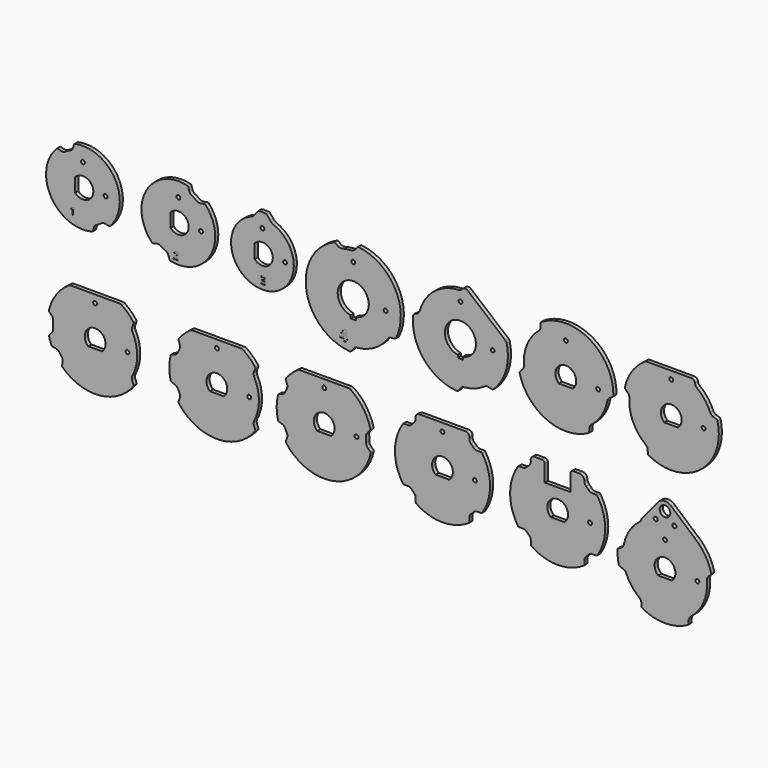
from build123d import *

# Parameters (mm, degrees)
F0_R           = 1.5
F1_DEPTH       = 1.5
F0_R_2         = 1.525
F0_R_3         = 4.1
F2_TEXT_SIZE   = 7.3750813802
F2_TEXT_SIZE_2 = 7.6333681742
F2_TEXT_SIZE_3 = 7.6956219143
F2_TEXT_SIZE_4 = 11.4732318454
F3_DEPTH       = 0.2


# Not quite as in the source:
# - ends of sketch curves that miss each other by under 0.0002 mm in the source are joined
# - Text() gives the source's letters only with a copy of the font that has no kerning and outlines rounded to 1/6400 em; it was checked with that copy


with BuildPart() as f1:
    # F0 (on Front) → F1 (new body, symmetric)
    with BuildSketch(Plane.XZ):
        with BuildLine():
            ThreePointArc((14200.079831, 8014.968847), (14199.2042357624, 8014.8382255006), (14198.4048882333, 8014.4577356533))
            ThreePointArc((14198.4048882333, 8014.4577356533), (14188.7422452749, 8004.9375996678), (14183.1913974519, 7992.5606958913))
            ThreePointArc((14183.1913974519, 7992.5606958913), (14183.196592645, 7992.0724746168), (14183.43232998, 7991.6449059814))
            Line((14183.43232998, 7991.6449059814), (14185.454349, 7989.476557))
            ThreePointArc((14185.454349, 7989.476557), (14186.3037649641, 7988.0716857602), (14186.5173174283, 7986.4439369673))
            ThreePointArc((14186.5173174283, 7986.4439369673), (14186.4232423777, 7983.8270392008), (14186.5401501982, 7981.2110620169))
            ThreePointArc((14186.5401501982, 7981.2110620169), (14186.3408101777, 7979.5815118733), (14185.5036861043, 7978.1692819044))
            Line((14185.5036861043, 7978.1692819044), (14183.500667, 7975.98337))
            ThreePointArc((14183.500667, 7975.98337), (14183.2686701473, 7975.5537602021), (14183.2677355957, 7975.0655121487))
            ThreePointArc((14183.2677355957, 7975.0655121487), (14184.1232508054, 7972.1559464606), (14185.2157560213, 7969.3268280092))
            ThreePointArc((14185.2157560213, 7969.3268280092), (14185.5137241497, 7968.9400433784), (14185.9593100369, 7968.7404422092))
            Line((14185.9593100369, 7968.7404422092), (14188.804696, 7968.238724))
            ThreePointArc((14188.804696, 7968.238724), (14190.2593014236, 7967.6730587895), (14191.3867109993, 7966.5937989995))
            Line((14191.3867109993, 7966.5937989995), (14192.282249, 7965.314839))
            Line((14192.282249, 7965.314839), (14193.177786, 7964.035879))
            ThreePointArc((14193.177786, 7964.035879), (14193.806362026, 7962.607331467), (14193.8404089622, 7961.0469800067))
            Line((14193.8404089622, 7961.0469800067), (14193.338691, 7958.201595))
            ThreePointArc((14193.338691, 7958.201595), (14193.3738547398, 7957.7146138253), (14193.6354021685, 7957.3023271776))
            ThreePointArc((14193.6354021685, 7957.3023271776), (14222.1259064772, 7947.3586918391), (14248.4568819619, 7962.0985850282))
            ThreePointArc((14248.4568819619, 7962.0985850282), (14248.6428628037, 7962.550025045), (14248.5929297112, 7963.0357138949))
            Line((14248.5929297112, 7963.0357138949), (14247.578894, 7965.821755))
            ThreePointArc((14247.578894, 7965.821755), (14247.3459288796, 7967.446839363), (14247.7853648796, 7969.0286320623))
            ThreePointArc((14247.7853648796, 7969.0286320623), (14251.422933, 7983.968847), (14247.7853649289, 7998.9090619632))
            ThreePointArc((14247.7853649289, 7998.9090619632), (14247.3459288906, 8000.4908544663), (14247.5788935935, 8002.115938784))
            Line((14247.5788935935, 8002.115938784), (14248.59293, 8004.90198))
            ThreePointArc((14248.59293, 8004.90198), (14248.6428628037, 8005.387668955), (14248.4568819968, 8005.8391089976))
            ThreePointArc((14248.4568819968, 8005.8391089976), (14244.3172375257, 8010.533707204), (14239.4409778247, 8014.4577357395))
            ThreePointArc((14239.4409778247, 8014.4577357395), (14238.6416302376, 8014.8382255006), (14237.766035, 8014.968847))
            Line((14237.766035, 8014.968847), (14200.079831, 8014.968847))
        make_face()
        with Locations((14243.922933, 7983.968847)):
            Circle(F0_R, mode=Mode.SUBTRACT)
        with BuildLine():
            ThreePointArc((14213.5787771393, 7977.9888471558), (14218.922933, 7991.988847), (14224.2670888607, 7977.9888471558))
            Line((14224.2670888607, 7977.9888471558), (14213.5787771393, 7977.9888471558))
        make_face(mode=Mode.SUBTRACT)
        with Locations((14218.922933, 8008.968847)):
            Circle(F0_R, mode=Mode.SUBTRACT)
    extrude(amount=F1_DEPTH, both=True)


with BuildPart() as f1b:
    # F0 (on Front) → F1, piece 2 (new body, symmetric)
    with BuildSketch(Plane.XZ):
        with BuildLine():
            ThreePointArc((14377.155191, 8014.968847), (14376.2795961592, 8014.8382256217), (14375.4802489216, 8014.4577361165))
            ThreePointArc((14375.4802489216, 8014.4577361165), (14370.6017890821, 8010.5316035955), (14366.4607222314, 8005.8342158287))
            ThreePointArc((14366.4607222314, 8005.8342158287), (14366.2748282895, 8005.3828269143), (14366.3247732888, 8004.8972201051))
            Line((14366.3247732888, 8004.8972201051), (14367.314353, 8002.17837))
            ThreePointArc((14367.314353, 8002.17837), (14367.5517758982, 8000.6358117234), (14367.1808141397, 7999.1198159349))
            Line((14367.1808141397, 7999.1198159349), (14366.520971, 7997.704778))
            Line((14366.520971, 7997.704778), (14365.861128, 7996.28974))
            ThreePointArc((14365.861128, 7996.28974), (14364.9382575593, 7995.0311034043), (14363.6039769009, 7994.2214422721))
            Line((14363.6039769009, 7994.2214422721), (14360.889031, 7993.233283))
            ThreePointArc((14360.889031, 7993.233283), (14360.4847933525, 7992.9592472118), (14360.258540747, 7992.5264500606))
            ThreePointArc((14360.258540747, 7992.5264500606), (14359.2482945731, 7983.9623568006), (14360.2615660243, 7975.3986210058))
            ThreePointArc((14360.2615660243, 7975.3986210058), (14360.4877361206, 7974.9661670482), (14360.8916420745, 7974.6922522044))
            Line((14360.8916420745, 7974.6922522044), (14363.605548, 7973.703386))
            ThreePointArc((14363.605548, 7973.703386), (14364.9395422638, 7972.893254628), (14365.8619682489, 7971.6342931159))
            Line((14365.8619682489, 7971.6342931159), (14366.521312, 7970.219022))
            Line((14366.521312, 7970.219022), (14367.180656, 7968.803751))
            ThreePointArc((14367.180656, 7968.803751), (14367.5510822042, 7967.2876244307), (14367.3131155041, 7965.7451501807))
            Line((14367.3131155041, 7965.7451501807), (14366.326797, 7963.038235))
            ThreePointArc((14366.326797, 7963.038235), (14366.2767123903, 7962.5524264045), (14366.4626788949, 7962.1008349222))
            ThreePointArc((14366.4626788949, 7962.1008349222), (14403.7875780239, 7948.0538145707), (14431.9395596858, 7976.3015188537))
            ThreePointArc((14431.9395596858, 7976.3015188537), (14431.9217192584, 7976.7896280066), (14431.6748163606, 7977.2110633544))
            Line((14431.6748163606, 7977.2110633544), (14429.691449, 7979.093208))
            ThreePointArc((14429.691449, 7979.093208), (14428.7283320504, 7980.5157322026), (14428.4507229301, 7982.2110500038))
            ThreePointArc((14428.4507229301, 7982.2110500038), (14428.4962942429, 7984.3293746859), (14428.4037393063, 7986.4461670234))
            ThreePointArc((14428.4037393063, 7986.4461670234), (14428.617224822, 7988.0740607591), (14429.4666868478, 7989.4790621419))
            Line((14429.4666868478, 7989.4790621419), (14431.488378, 7991.64706))
            ThreePointArc((14431.488378, 7991.64706), (14431.7241230993, 7992.0746590546), (14431.7292962492, 7992.5629108194))
            ThreePointArc((14431.7292962492, 7992.5629108194), (14426.1783315207, 8004.9385354872), (14416.5163381364, 8014.4577362027))
            ThreePointArc((14416.5163381364, 8014.4577362027), (14415.7169908408, 8014.8382256217), (14414.841396, 8014.968847))
            Line((14414.841396, 8014.968847), (14377.155191, 8014.968847))
        make_face()
        with BuildLine():
            ThreePointArc((14390.6541381393, 7977.9888471558), (14395.9982943728, 7991.988847), (14401.3424493048, 7977.988846659))
            Line((14401.3424493048, 7977.988846659), (14390.6541381393, 7977.9888471558))
        make_face(mode=Mode.SUBTRACT)
        with Locations((14420.998294, 7983.968847)):
            Circle(F0_R, mode=Mode.SUBTRACT)
        with Locations((14395.998294, 8008.968847)):
            Circle(F0_R, mode=Mode.SUBTRACT)
    extrude(amount=F1_DEPTH, both=True)


with BuildPart() as f1c:
    # F0 (on Front) → F1, piece 3 (new body, symmetric)
    with BuildSketch(Plane.XZ):
        with BuildLine():
            ThreePointArc((14351.617627481, 8112.5891055645), (14351.3167517551, 8112.8315400226), (14350.9464260229, 8112.9418102406))
            ThreePointArc((14350.9464260229, 8112.9418102406), (14348.2432924977, 8113.070286), (14345.5401589558, 8112.9418104636))
            ThreePointArc((14345.5401589558, 8112.9418104636), (14345.16983297, 8112.8315404036), (14344.8689569322, 8112.5891060569))
            Line((14344.8689569322, 8112.5891060569), (14341.39996, 8108.454916))
            ThreePointArc((14341.39996, 8108.454916), (14340.6452085072, 8107.7600986585), (14339.7385518917, 8107.2801042892))
            ThreePointArc((14339.7385518917, 8107.2801042892), (14348.2432915318, 8060.317728), (14356.7480329039, 8107.2801037435))
            ThreePointArc((14356.7480329039, 8107.2801037435), (14355.8413758751, 8107.7600983882), (14355.0866244099, 8108.4549163439))
            Line((14355.0866244099, 8108.4549163439), (14351.617627481, 8112.5891055645))
        make_face()
        with BuildLine():
            ThreePointArc((14342.2632921558, 8089.9131628607), (14356.263292, 8084.569007), (14342.2632921558, 8079.2248511393))
            Line((14342.2632921558, 8079.2248511393), (14342.2632921558, 8089.9131628607))
        make_face(mode=Mode.SUBTRACT)
        with Locations((14365.743292, 8084.569007)):
            Circle(F0_R, mode=Mode.SUBTRACT)
        with Locations((14348.243292, 8102.069007)):
            Circle(F0_R, mode=Mode.SUBTRACT)
    extrude(amount=F1_DEPTH, both=True)


with BuildPart() as f1d:
    # F0 (on Front) → F1, piece 4 (new body, symmetric)
    with BuildSketch(Plane.XZ):
        with BuildLine():
            ThreePointArc((14269.6530267605, 8064.4850036461), (14271.4866589172, 8063.3594789865), (14273.4128349841, 8062.4009079642))
            ThreePointArc((14273.4128349841, 8062.4009079642), (14274.761907334, 8061.42304264), (14275.5955420523, 8059.980382017))
            Line((14275.5955420523, 8059.980382017), (14276.437028, 8057.390555))
            ThreePointArc((14276.437028, 8057.390555), (14276.7170541628, 8056.9581425593), (14277.1751681478, 8056.7225016781))
            ThreePointArc((14277.1751681478, 8056.7225016781), (14307.9250160099, 8070.3190070035), (14304.325011269, 8103.7474092447))
            ThreePointArc((14304.325011269, 8103.7474092447), (14303.8918832817, 8104.0263274819), (14303.3773898912, 8104.0526305119))
            Line((14303.3773898912, 8104.0526305119), (14300.713791, 8103.486465))
            ThreePointArc((14300.713791, 8103.486465), (14299.0475925223, 8103.4870831403), (14297.5262000244, 8104.1664820335))
            ThreePointArc((14297.5262000244, 8104.1664820335), (14295.732965508, 8105.355313927), (14293.8414167535, 8106.3805234927))
            ThreePointArc((14293.8414167535, 8106.3805234927), (14292.5272932377, 8107.4048750153), (14291.7445143526, 8108.8757501011))
            Line((14291.7445143526, 8108.8757501011), (14290.993924, 8111.493367))
            ThreePointArc((14290.993924, 8111.493367), (14290.729160386, 8111.9352893295), (14290.2795488878, 8112.1867745596))
            ThreePointArc((14290.2795488878, 8112.1867745596), (14258.5615680154, 8098.8190070404), (14262.8437320257, 8064.6665460251))
            ThreePointArc((14262.8437320257, 8064.6665460251), (14263.2863302104, 8064.4029138697), (14263.8014279296, 8064.3945822822))
            Line((14263.8014279296, 8064.3945822822), (14266.443646, 8065.053361))
            ThreePointArc((14266.443646, 8065.053361), (14268.1088506854, 8065.1108923173), (14269.6530267605, 8064.4850036461))
        make_face()
        with BuildLine():
            ThreePointArc((14277.2632921558, 8089.9131628607), (14291.263292, 8084.569007), (14277.2632921558, 8079.2248511393))
            Line((14277.2632921558, 8079.2248511393), (14277.2632921558, 8089.9131628607))
        make_face(mode=Mode.SUBTRACT)
        with Locations((14300.743292, 8084.569007)):
            Circle(F0_R, mode=Mode.SUBTRACT)
        with Locations((14283.243292, 8102.069007)):
            Circle(F0_R, mode=Mode.SUBTRACT)
    extrude(amount=F1_DEPTH, both=True)


with BuildPart() as f1e:
    # F0 (on Front) → F1, piece 5 (new body, symmetric)
    with BuildSketch(Plane.XZ):
        with BuildLine():
            ThreePointArc((14465.2632651508, 8081.5638557103), (14464.8983238973, 8081.2395025105), (14464.7304549139, 8080.781019009))
            ThreePointArc((14464.7304549139, 8080.781019009), (14473.1283676669, 8053.3301764018), (14498.7038879942, 8040.2930579173))
            ThreePointArc((14498.7038879942, 8040.2930579173), (14499.1845564273, 8040.3787618066), (14499.5673534214, 8040.6818356767))
            Line((14499.5673534214, 8040.6818356767), (14501.372236, 8043.034004))
            ThreePointArc((14501.372236, 8043.034004), (14502.6176457488, 8044.103641076), (14504.1878239991, 8044.5829210105))
            ThreePointArc((14504.1878239991, 8044.5829210105), (14512.3961554837, 8046.412610761), (14519.8602041113, 8050.2872008403))
            ThreePointArc((14519.8602041113, 8050.2872008403), (14521.3711059469, 8050.9293425229), (14523.0126950274, 8050.9104871235))
            Line((14523.0126950274, 8050.9104871235), (14525.907259, 8050.268778))
            ThreePointArc((14525.907259, 8050.268778), (14526.3953106024, 8050.28266705), (14526.8186134441, 8050.5259815752))
            ThreePointArc((14526.8186134441, 8050.5259815752), (14536.5308057411, 8066.5613498719), (14537.0697366746, 8085.3008609241))
            ThreePointArc((14537.0697366746, 8085.3008609241), (14536.7043053022, 8086.1897706333), (14536.0765290915, 8086.9175051091))
            Line((14536.0765290915, 8086.9175051091), (14506.988961, 8111.324873))
            ThreePointArc((14506.988961, 8111.324873), (14504.7991311131, 8112.0153241241), (14502.7624648909, 8110.9551030915))
            Line((14502.7624648909, 8110.9551030915), (14502.668363, 8110.842957))
            ThreePointArc((14502.668363, 8110.842957), (14501.3774813305, 8109.8286614037), (14499.7878910131, 8109.4183277142))
            ThreePointArc((14499.7878910131, 8109.4183277142), (14480.9379880698, 8102.2988666329), (14469.9074209954, 8085.4367150013))
            ThreePointArc((14469.9074209954, 8085.4367150013), (14469.1627633768, 8083.9736170775), (14467.8931128233, 8082.9328683395))
            Line((14467.8931128233, 8082.9328683395), (14465.2632651508, 8081.5638557103))
        make_face()
        with BuildLine():
            ThreePointArc((14499.1066709815, 8065.1308248991), (14501.280501, 8088.972621), (14503.4543310185, 8065.1308248991))
            ThreePointArc((14503.4543310185, 8065.1308248991), (14503.3368227567, 8065.0621190841), (14503.290501, 8064.934123))
            Line((14503.290501, 8064.934123), (14503.290501, 8062.932621))
            Line((14503.290501, 8062.932621), (14499.270501, 8062.932621))
            Line((14499.270501, 8062.932621), (14499.270501, 8064.934123))
            ThreePointArc((14499.270501, 8064.934123), (14499.2241792433, 8065.0621190841), (14499.1066709815, 8065.1308248991))
        make_face(mode=Mode.SUBTRACT)
        with Locations((14526.280501, 8076.952621)):
            Circle(F0_R, mode=Mode.SUBTRACT)
        with Locations((14501.280501, 8101.952621)):
            Circle(F0_R, mode=Mode.SUBTRACT)
    extrude(amount=F1_DEPTH, both=True)


with BuildPart() as f1f:
    # F0 (on Front) → F1, piece 6 (new body, symmetric)
    with BuildSketch(Plane.XZ):
        with BuildLine():
            ThreePointArc((14419.8450266694, 8110.8429564384), (14418.5541445947, 8109.8286610398), (14416.9645540152, 8109.4183276683))
            ThreePointArc((14416.9645540152, 8109.4183276683), (14413.5131538397, 8109.0743700734), (14410.1180649261, 8108.3645522784))
            ThreePointArc((14410.1180649261, 8108.3645522784), (14408.4786560745, 8108.2778953364), (14406.9425158086, 8108.8570706996))
            Line((14406.9425158086, 8108.8570706996), (14404.441993, 8110.45008))
            ThreePointArc((14404.441993, 8110.45008), (14403.9786240025, 8110.6039513588), (14403.4976311748, 8110.5200886079))
            ThreePointArc((14403.4976311748, 8110.5200886079), (14382.2654791211, 8070.5710502193), (14415.8805519893, 8040.2930578473))
            ThreePointArc((14415.8805519893, 8040.2930578473), (14416.3612204273, 8040.3787618066), (14416.7440174214, 8040.6818356767))
            Line((14416.7440174214, 8040.6818356767), (14418.548899, 8043.034004))
            ThreePointArc((14418.548899, 8043.034004), (14419.7943091851, 8044.103641316), (14421.3644879911, 8044.5829210996))
            ThreePointArc((14421.3644879911, 8044.5829210996), (14434.7071642776, 8048.8067955373), (14445.0364847442, 8058.24995518))
            ThreePointArc((14445.0364847442, 8058.24995518), (14446.236642671, 8059.370130103), (14447.7856809463, 8059.913868408))
            Line((14447.7856809463, 8059.913868408), (14450.72516, 8060.300858))
            ThreePointArc((14450.72516, 8060.300858), (14451.1790276572, 8060.4808334167), (14451.4935832903, 8060.8542523458))
            ThreePointArc((14451.4935832903, 8060.8542523458), (14450.6768720866, 8094.6289585961), (14422.6303920065, 8113.4649020573))
            ThreePointArc((14422.6303920065, 8113.4649020573), (14422.1464428756, 8113.400246489), (14421.7507904398, 8113.1141584701))
            Line((14421.7507904398, 8113.1141584701), (14419.8450266694, 8110.8429564384))
        make_face()
        with BuildLine():
            ThreePointArc((14416.447164, 8064.934123), (14416.400842558, 8065.0621187062), (14416.2833349918, 8065.1308249556))
            ThreePointArc((14416.2833349918, 8065.1308249556), (14418.4571635083, 8088.972621), (14420.6309940185, 8065.1308248991))
            ThreePointArc((14420.6309940185, 8065.1308248991), (14420.5134857567, 8065.0621190841), (14420.467164, 8064.934123))
            Line((14420.467164, 8064.934123), (14420.467164, 8062.932621))
            Line((14420.467164, 8062.932621), (14416.447164, 8062.932621))
            Line((14416.447164, 8062.932621), (14416.447164, 8064.934123))
        make_face(mode=Mode.SUBTRACT)
        with Locations((14418.457164, 8101.952621)):
            Circle(F0_R, mode=Mode.SUBTRACT)
        with Locations((14443.457164, 8076.952621)):
            Circle(F0_R, mode=Mode.SUBTRACT)
    extrude(amount=F1_DEPTH, both=True)


with BuildPart() as f1g:
    # F0 (on Front) → F1, piece 7 (new body, symmetric)
    with BuildSketch(Plane.XZ):
        with BuildLine():
            ThreePointArc((14333.5544847667, 8014.4577356533), (14332.7551372376, 8014.8382255006), (14331.879542, 8014.968847))
            Line((14331.879542, 8014.968847), (14294.193338, 8014.968847))
            ThreePointArc((14294.193338, 8014.968847), (14293.3177431592, 8014.8382256217), (14292.5183959216, 8014.4577361165))
            ThreePointArc((14292.5183959216, 8014.4577361165), (14287.6399355969, 8010.5316040878), (14283.4988685854, 8005.8342163069))
            ThreePointArc((14283.4988685854, 8005.8342163069), (14283.3129743077, 8005.3828270394), (14283.3629194058, 8004.8972197837))
            Line((14283.3629194058, 8004.8972197837), (14284.3525, 8002.17837))
            ThreePointArc((14284.3525, 8002.17837), (14284.5899228982, 8000.6358117234), (14284.2189611397, 7999.1198159349))
            Line((14284.2189611397, 7999.1198159349), (14283.559118, 7997.704778))
            Line((14283.559118, 7997.704778), (14282.899274, 7996.28974))
            ThreePointArc((14282.899274, 7996.28974), (14281.9764039057, 7995.0311037217), (14280.642123784, 7994.2214425935))
            Line((14280.642123784, 7994.2214425935), (14277.927178, 7993.233283))
            ThreePointArc((14277.927178, 7993.233283), (14277.5229403525, 7992.9592472118), (14277.296687747, 7992.5264500606))
            ThreePointArc((14277.296687747, 7992.5264500606), (14276.2864405731, 7983.962356917), (14277.2997120243, 7975.3986210058))
            ThreePointArc((14277.2997120243, 7975.3986210058), (14277.5258824333, 7974.9661666976), (14277.9297889573, 7974.6922518827))
            Line((14277.9297889573, 7974.6922518827), (14280.643695, 7973.703386))
            ThreePointArc((14280.643695, 7973.703386), (14281.9776892638, 7972.893254628), (14282.9001152489, 7971.6342931159))
            Line((14282.9001152489, 7971.6342931159), (14283.559459, 7970.219022))
            Line((14283.559459, 7970.219022), (14284.218802, 7968.803751))
            ThreePointArc((14284.218802, 7968.803751), (14284.5892292025, 7967.2876244706), (14284.3512623869, 7965.745149859))
            Line((14284.3512623869, 7965.745149859), (14283.364944, 7963.038235))
            ThreePointArc((14283.364944, 7963.038235), (14283.3148593476, 7962.5524266989), (14283.5008255408, 7962.1008354004))
            ThreePointArc((14283.5008255408, 7962.1008354004), (14313.0350401736, 7947.2188470267), (14342.5703889619, 7962.0985850282))
            ThreePointArc((14342.5703889619, 7962.0985850282), (14342.7563698037, 7962.550025045), (14342.7064367112, 7963.0357138949))
            Line((14342.7064367112, 7963.0357138949), (14341.692401, 7965.821755))
            ThreePointArc((14341.692401, 7965.821755), (14341.4594358796, 7967.446839363), (14341.8988718796, 7969.0286320623))
            ThreePointArc((14341.8988718796, 7969.0286320623), (14345.53644, 7983.968847), (14341.8988719289, 7998.9090619632))
            ThreePointArc((14341.8988719289, 7998.9090619632), (14341.4594358796, 8000.490854637), (14341.6924007105, 8002.1159391054))
            Line((14341.6924007105, 8002.1159391054), (14342.706437, 8004.90198))
            ThreePointArc((14342.706437, 8004.90198), (14342.7563698037, 8005.387668955), (14342.5703889968, 8005.8391089976))
            ThreePointArc((14342.5703889968, 8005.8391089976), (14338.4307445257, 8010.533707204), (14333.5544847667, 8014.4577356533))
        make_face()
        with Locations((14338.03644, 7983.968847)):
            Circle(F0_R, mode=Mode.SUBTRACT)
        with BuildLine():
            ThreePointArc((14307.6922846952, 7977.988846659), (14313.0364396272, 7991.988847), (14318.3805958607, 7977.9888471558))
            Line((14318.3805958607, 7977.9888471558), (14307.6922846952, 7977.988846659))
        make_face(mode=Mode.SUBTRACT)
        with Locations((14313.03644, 8008.968847)):
            Circle(F0_R, mode=Mode.SUBTRACT)
    extrude(amount=F1_DEPTH, both=True)


with BuildPart() as f1h:
    # F0 (on Front) → F1, piece 8 (new body, symmetric)
    with BuildSketch(Plane.XZ):
        with BuildLine():
            ThreePointArc((14514.305271, 8004.689971), (14512.6985127496, 8005.0268674081), (14511.3624100409, 8005.9808070376))
            ThreePointArc((14511.3624100409, 8005.9808070376), (14510.4326373886, 8006.9498173886), (14509.4636268557, 8007.8795898432))
            ThreePointArc((14509.4636268557, 8007.8795898432), (14508.3900564081, 8009.5220975838), (14508.2267972941, 8011.4775339512))
            ThreePointArc((14508.2267972941, 8011.4775339512), (14507.5557446006, 8013.9087002068), (14505.267302, 8014.968847))
            Line((14505.267302, 8014.968847), (14469.636032, 8014.968847))
            ThreePointArc((14469.636032, 8014.968847), (14467.3475893994, 8013.9087002068), (14466.6765368551, 8011.477533976))
            ThreePointArc((14466.6765368551, 8011.477533976), (14466.5132775919, 8009.5220975838), (14465.4397069624, 8007.8795900409))
            ThreePointArc((14465.4397069624, 8007.8795900409), (14464.4706966114, 8006.9498173886), (14463.5409241568, 8005.9808068556))
            ThreePointArc((14463.5409241568, 8005.9808068556), (14462.2048212504, 8005.0268674081), (14460.598063, 8004.689971))
            Line((14460.598063, 8004.689971), (14457.63322, 8004.689971))
            ThreePointArc((14457.63322, 8004.689971), (14457.1597435727, 8004.57077749), (14456.7991377799, 8004.2416111455))
            ThreePointArc((14456.7991377799, 8004.2416111455), (14450.701667, 7983.968847), (14456.7991379353, 7963.6960829572))
            ThreePointArc((14456.7991379353, 7963.6960829572), (14457.1597435727, 7963.36691651), (14457.63322, 7963.247723))
            Line((14457.63322, 7963.247723), (14460.598063, 7963.247723))
            ThreePointArc((14460.598063, 7963.247723), (14462.2048212504, 7962.9108265919), (14463.5409239591, 7961.9568869624))
            ThreePointArc((14463.5409239591, 7961.9568869624), (14464.4706966114, 7960.9878766114), (14465.4397071444, 7960.0581041568))
            ThreePointArc((14465.4397071444, 7960.0581041568), (14466.3936465919, 7958.7220012504), (14466.730543, 7957.115243))
            Line((14466.730543, 7957.115243), (14466.730543, 7954.1504))
            ThreePointArc((14466.730543, 7954.1504), (14466.84973651, 7953.6769235727), (14467.1789028545, 7953.3163177799))
            ThreePointArc((14467.1789028545, 7953.3163177799), (14487.451667, 7947.218847), (14507.7244310428, 7953.3163179353))
            ThreePointArc((14507.7244310428, 7953.3163179353), (14508.05359749, 7953.6769235727), (14508.172791, 7954.1504))
            Line((14508.172791, 7954.1504), (14508.172791, 7957.115243))
            ThreePointArc((14508.172791, 7957.115243), (14508.5096874081, 7958.7220012504), (14509.4636270376, 7960.0581039591))
            ThreePointArc((14509.4636270376, 7960.0581039591), (14510.4326373886, 7960.9878766114), (14511.3624098432, 7961.9568871444))
            ThreePointArc((14511.3624098432, 7961.9568871444), (14512.6985127496, 7962.9108265919), (14514.305271, 7963.247723))
            Line((14514.305271, 7963.247723), (14517.270114, 7963.247723))
            ThreePointArc((14517.270114, 7963.247723), (14517.7435904273, 7963.36691651), (14518.1041962201, 7963.6960828545))
            ThreePointArc((14518.1041962201, 7963.6960828545), (14524.201667, 7983.968847), (14518.1041960647, 8004.2416110428))
            ThreePointArc((14518.1041960647, 8004.2416110428), (14517.7435904273, 8004.57077749), (14517.270114, 8004.689971))
            Line((14517.270114, 8004.689971), (14514.305271, 8004.689971))
        make_face()
        with BuildLine():
            ThreePointArc((14482.1075111393, 7977.9888471558), (14487.451667, 7991.988847), (14492.7958228607, 7977.9888471558))
            Line((14492.7958228607, 7977.9888471558), (14482.1075111393, 7977.9888471558))
        make_face(mode=Mode.SUBTRACT)
        with Locations((14512.451667, 7983.968847)):
            Circle(F0_R, mode=Mode.SUBTRACT)
        with Locations((14487.451667, 8008.968847)):
            Circle(F0_R, mode=Mode.SUBTRACT)
    extrude(amount=F1_DEPTH, both=True)


with BuildPart() as f1i:
    # F0 (on Front) → F1, piece 9 (new body, symmetric)
    with BuildSketch(Plane.XZ):
        with BuildLine():
            ThreePointArc((14555.6802867059, 8011.4775339512), (14555.5170275919, 8009.5220975838), (14554.4434569624, 8007.8795900409))
            ThreePointArc((14554.4434569624, 8007.8795900409), (14553.4744466114, 8006.9498173886), (14552.5446741568, 8005.9808068556))
            ThreePointArc((14552.5446741568, 8005.9808068556), (14551.2085712504, 8005.0268674081), (14549.601813, 8004.689971))
            Line((14549.601813, 8004.689971), (14546.63697, 8004.689971))
            ThreePointArc((14546.63697, 8004.689971), (14546.1634935727, 8004.57077749), (14545.8028877799, 8004.2416111455))
            ThreePointArc((14545.8028877799, 8004.2416111455), (14539.705417, 7983.968847), (14545.8028879353, 7963.6960829572))
            ThreePointArc((14545.8028879353, 7963.6960829572), (14546.1634935727, 7963.36691651), (14546.63697, 7963.247723))
            Line((14546.63697, 7963.247723), (14549.601813, 7963.247723))
            ThreePointArc((14549.601813, 7963.247723), (14551.2085712504, 7962.9108265919), (14552.5446739591, 7961.9568869624))
            ThreePointArc((14552.5446739591, 7961.9568869624), (14553.4744466114, 7960.9878766114), (14554.4434571444, 7960.0581041568))
            ThreePointArc((14554.4434571444, 7960.0581041568), (14555.3973965919, 7958.7220012504), (14555.734293, 7957.115243))
            Line((14555.734293, 7957.115243), (14555.734293, 7954.1504))
            ThreePointArc((14555.734293, 7954.1504), (14555.85348651, 7953.6769235727), (14556.1826528545, 7953.3163177799))
            ThreePointArc((14556.1826528545, 7953.3163177799), (14576.455417, 7947.218847), (14596.7281810428, 7953.3163179353))
            ThreePointArc((14596.7281810428, 7953.3163179353), (14597.05734749, 7953.6769235727), (14597.176541, 7954.1504))
            Line((14597.176541, 7954.1504), (14597.176541, 7957.115243))
            ThreePointArc((14597.176541, 7957.115243), (14597.5134372604, 7958.7220009135), (14598.4673764963, 7960.0581034609))
            ThreePointArc((14598.4673764963, 7960.0581034609), (14599.4363871285, 7960.9878763513), (14600.3661598432, 7961.9568871444))
            ThreePointArc((14600.3661598432, 7961.9568871444), (14601.7022627496, 7962.9108265919), (14603.309021, 7963.247723))
            Line((14603.309021, 7963.247723), (14606.273864, 7963.247723))
            ThreePointArc((14606.273864, 7963.247723), (14606.7473404273, 7963.36691651), (14607.1079462201, 7963.6960828545))
            ThreePointArc((14607.1079462201, 7963.6960828545), (14613.205417, 7983.968847), (14607.1079460647, 8004.2416110428))
            ThreePointArc((14607.1079460647, 8004.2416110428), (14606.7473404273, 8004.57077749), (14606.273864, 8004.689971))
            Line((14606.273864, 8004.689971), (14603.309021, 8004.689971))
            ThreePointArc((14603.309021, 8004.689971), (14601.7022627496, 8005.0268674081), (14600.3661600409, 8005.9808070376))
            ThreePointArc((14600.3661600409, 8005.9808070376), (14599.4363871285, 8006.9498176487), (14598.4673763144, 8007.8795903415))
            ThreePointArc((14598.4673763144, 8007.8795903415), (14597.4988885607, 8009.249278239), (14597.1772107995, 8010.8956490037))
            ThreePointArc((14597.1772107995, 8010.8956490037), (14596.0320691967, 8013.771275238), (14593.17788, 8014.968847))
            Line((14593.17788, 8014.968847), (14588.455417, 8014.968847))
            ThreePointArc((14588.455417, 8014.968847), (14587.0412034376, 8014.3830605624), (14586.455417, 8012.968847))
            Line((14586.455417, 8012.968847), (14586.455417, 8000.168847))
            ThreePointArc((14586.455417, 8000.168847), (14586.3968383562, 8000.0274256438), (14586.255417, 7999.968847))
            Line((14586.255417, 7999.968847), (14566.655417, 7999.968847))
            ThreePointArc((14566.655417, 7999.968847), (14566.5139956438, 8000.0274256438), (14566.455417, 8000.168847))
            Line((14566.455417, 8000.168847), (14566.455417, 8012.968847))
            ThreePointArc((14566.455417, 8012.968847), (14565.8696305624, 8014.3830605624), (14564.455417, 8014.968847))
            Line((14564.455417, 8014.968847), (14558.639782, 8014.968847))
            ThreePointArc((14558.639782, 8014.968847), (14556.3513393994, 8013.9087002068), (14555.6802867059, 8011.4775339512))
        make_face()
        with Locations((14601.455417, 7983.968847)):
            Circle(F0_R, mode=Mode.SUBTRACT)
        with BuildLine():
            ThreePointArc((14571.1112611393, 7977.9888471558), (14576.455417, 7991.988847), (14581.7995728607, 7977.9888471558))
            Line((14581.7995728607, 7977.9888471558), (14571.1112611393, 7977.9888471558))
        make_face(mode=Mode.SUBTRACT)
    extrude(amount=F1_DEPTH, both=True)


with BuildPart() as f1j:
    # F0 (on Front) → F1, piece 10 (new body, symmetric)
    with BuildSketch(Plane.XZ):
        with BuildLine():
            ThreePointArc((14677.7596142086, 7942.6995559818), (14678.2352894013, 7944.2708788152), (14679.3020999258, 7945.5187720962))
            ThreePointArc((14679.3020999258, 7945.5187720962), (14689.2055315851, 7958.1669248516), (14691.8414227449, 7974.0132429783))
            ThreePointArc((14691.8414227449, 7974.0132429783), (14692.0408236399, 7975.6426639762), (14692.8779078957, 7977.0547770956))
            Line((14692.8779078957, 7977.0547770956), (14694.881218, 7979.241007))
            ThreePointArc((14694.881218, 7979.241007), (14695.113208819, 7979.6705890832), (14695.1141640936, 7980.1588100234))
            ThreePointArc((14695.1141640936, 7980.1588100234), (14690.3876938836, 7991.1055275704), (14682.4053861559, 7999.9628921951))
            Line((14682.4053861559, 7999.9628921951), (14664.650409, 8015.400468))
            ThreePointArc((14664.650409, 8015.400468), (14659.3018076709, 8017.7036357253), (14654.0616295503, 8015.1634293715))
            Line((14654.0616295503, 8015.1634293715), (14641.454524, 7999.901448))
            ThreePointArc((14641.454524, 7999.901448), (14641.3031813508, 7999.6837717845), (14641.21435795, 7999.4339760106))
            ThreePointArc((14641.21435795, 7999.4339760106), (14640.6825552245, 7998.1258537481), (14639.7293447838, 7997.084034283))
            ThreePointArc((14639.7293447838, 7997.084034283), (14631.8763793461, 7988.4469491314), (14627.5818186098, 7977.5922240775))
            ThreePointArc((14627.5818186098, 7977.5922240775), (14626.8480367672, 7975.9579464827), (14625.4745010389, 7974.8078599236))
            Line((14625.4745010389, 7974.8078599236), (14623.28789, 7973.693726))
            ThreePointArc((14623.28789, 7973.693726), (14622.9007347635, 7973.3435277374), (14622.7428155927, 7972.8459439744))
            ThreePointArc((14622.7428155927, 7972.8459439744), (14622.8777283907, 7967.7344110086), (14623.7208198794, 7962.6910819711))
            ThreePointArc((14623.7208198794, 7962.6910819711), (14623.9470966976, 7962.2584316048), (14624.3512527837, 7961.9844874058))
            Line((14624.3512527837, 7961.9844874058), (14627.137294, 7960.970452))
            ThreePointArc((14627.137294, 7960.970452), (14628.5319276615, 7960.1043291335), (14629.4611871968, 7958.750945082))
            ThreePointArc((14629.4611871968, 7958.750945082), (14633.6744858284, 7951.4727190517), (14639.6142304475, 7945.5192415804))
            ThreePointArc((14639.6142304475, 7945.5192415804), (14640.6809891413, 7944.2713646133), (14641.1566417838, 7942.7000830686))
            Line((14641.1566417838, 7942.7000830686), (14641.415044, 7939.746522))
            ThreePointArc((14641.415044, 7939.746522), (14641.5750507364, 7939.2852354891), (14641.9343938332, 7938.9546906924))
            ThreePointArc((14641.9343938332, 7938.9546906924), (14659.4580778978, 7934.5074660021), (14676.9818565957, 7938.9543177452))
            ThreePointArc((14676.9818565957, 7938.9543177452), (14677.3412124865, 7939.2848636811), (14677.501224678, 7939.7461590282))
            Line((14677.501224678, 7939.7461590282), (14677.7596142086, 7942.6995559818))
        make_face()
        with BuildLine():
            ThreePointArc((14654.1143136952, 7965.277465659), (14659.4584686272, 7979.277466), (14664.8026248607, 7965.2774661558))
            Line((14664.8026248607, 7965.2774661558), (14654.1143136952, 7965.277465659))
        make_face(mode=Mode.SUBTRACT)
        with Locations((14684.458469, 7971.257466)):
            Circle(F0_R, mode=Mode.SUBTRACT)
        with Locations((14659.458469, 7991.257466)):
            Circle(F0_R, mode=Mode.SUBTRACT)
        with Locations((14652.167551, 8003.072707)):
            Circle(F0_R_2, mode=Mode.SUBTRACT)
        with Locations((14666.749388, 8003.072707)):
            Circle(F0_R_2, mode=Mode.SUBTRACT)
        with Locations((14659.458469, 8010.705389)):
            Circle(F0_R_3, mode=Mode.SUBTRACT)
    extrude(amount=F1_DEPTH, both=True)


with BuildPart() as f1k:
    # F0 (on Front) → F1, piece 11 (new body, symmetric)
    with BuildSketch(Plane.XZ):
        with BuildLine():
            ThreePointArc((14631.8563672315, 8078.8593240451), (14634.7274562282, 8063.4761399152), (14644.4548939672, 8051.2179809574))
            ThreePointArc((14644.4548939672, 8051.2179809574), (14645.52153253, 8049.9701418563), (14645.9971327914, 8048.3989559818))
            Line((14645.9971327914, 8048.3989559818), (14646.255636, 8045.444248))
            ThreePointArc((14646.255636, 8045.444248), (14646.4156009929, 8044.983024139), (14646.7748529022, 8044.6524878197))
            ThreePointArc((14646.7748529022, 8044.6524878197), (14686.6739350194, 8047.7954697377), (14700.04124024, 8085.5198680575))
            ThreePointArc((14700.04124024, 8085.5198680575), (14699.814960954, 8085.952503752), (14699.4108128949, 8086.2264387112))
            Line((14699.4108128949, 8086.2264387112), (14696.62198, 8087.241491))
            ThreePointArc((14696.62198, 8087.241491), (14695.2273190056, 8088.107639927), (14694.2980581434, 8089.4610680598))
            ThreePointArc((14694.2980581434, 8089.4610680598), (14690.0865983702, 8096.7371596857), (14684.1496906641, 8102.6895565646))
            ThreePointArc((14684.1496906641, 8102.6895565646), (14683.1243500031, 8103.8641858684), (14682.6259925566, 8105.3415879424))
            ThreePointArc((14682.6259925566, 8105.3415879424), (14681.6309647836, 8107.2089420708), (14679.650989, 8107.955124))
            Line((14679.650989, 8107.955124), (14645.450069, 8107.955124))
            ThreePointArc((14645.450069, 8107.955124), (14644.5742147219, 8107.8244234412), (14643.7746768728, 8107.443710189))
            ThreePointArc((14643.7746768728, 8107.443710189), (14633.9321042931, 8097.6583403035), (14628.4199887626, 8084.9207470527))
            ThreePointArc((14628.4199887626, 8084.9207470527), (14628.4337258535, 8084.4327211005), (14628.6768814008, 8084.0093614213))
            Line((14628.6768814008, 8084.0093614213), (14630.740598, 8081.87232))
            ThreePointArc((14630.740598, 8081.87232), (14631.614297111, 8080.4827741274), (14631.8563672315, 8078.8593240451))
        make_face()
        with BuildLine():
            ThreePointArc((14658.9563796952, 8070.975123659), (14664.3005346272, 8084.975124), (14669.6446908607, 8070.9751241558))
            Line((14669.6446908607, 8070.9751241558), (14658.9563796952, 8070.975123659))
        make_face(mode=Mode.SUBTRACT)
        with Locations((14689.303798, 8076.952621)):
            Circle(F0_R, mode=Mode.SUBTRACT)
        with Locations((14664.303798, 8101.952621)):
            Circle(F0_R, mode=Mode.SUBTRACT)
    extrude(amount=F1_DEPTH, both=True)


with BuildPart() as f1l:
    # F0 (on Front) → F1, piece 12 (new body, symmetric)
    with BuildSketch(Plane.XZ):
        with BuildLine():
            ThreePointArc((14601.0932942086, 8048.3947119818), (14601.5689694013, 8049.9660348152), (14602.6357799258, 8051.2139280962))
            ThreePointArc((14602.6357799258, 8051.2139280962), (14610.576063271, 8060.0913011293), (14614.7849280974, 8071.2331729826))
            ThreePointArc((14614.7849280974, 8071.2331729826), (14615.3992599038, 8072.7554639486), (14616.5733029731, 8073.9028070422))
            Line((14616.5733029731, 8073.9028070422), (14619.07419, 8075.496048))
            ThreePointArc((14619.07419, 8075.496048), (14619.4094595403, 8075.8509490848), (14619.5367428937, 8076.3222870018))
            ThreePointArc((14619.5367428937, 8076.3222870018), (14601.1671491275, 8108.7790545155), (14563.8739670599, 8108.4592059003))
            ThreePointArc((14563.8739670599, 8108.4592059003), (14563.5294181927, 8108.1133058242), (14563.3896997601, 8107.6455029668))
            Line((14563.3896997601, 8107.6455029668), (14563.260356, 8104.683051))
            ThreePointArc((14563.260356, 8104.683051), (14562.853748781, 8103.0926284587), (14561.8425717225, 8101.7994563292))
            ThreePointArc((14561.8425717225, 8101.7994563292), (14552.8200794482, 8089.5194442574), (14550.3865918069, 8074.4767649852))
            ThreePointArc((14550.3865918069, 8074.4767649852), (14550.1730625536, 8072.8489667169), (14549.3236311161, 8071.4440508918))
            Line((14549.3236311161, 8071.4440508918), (14547.301725, 8069.275822))
            ThreePointArc((14547.301725, 8069.275822), (14547.0659848989, 8068.8482429449), (14547.0607973921, 8068.3600110943))
            ThreePointArc((14547.0607973921, 8068.3600110943), (14567.8445774708, 8043.3798253854), (14600.3155370149, 8044.6494729726))
            ThreePointArc((14600.3155370149, 8044.6494729726), (14600.6748928905, 8044.980019297), (14600.8349047649, 8045.4413150206))
            Line((14600.8349047649, 8045.4413150206), (14601.0932942086, 8048.3947119818))
        make_face()
        with BuildLine():
            ThreePointArc((14577.4479936952, 8070.972620659), (14582.7921486272, 8084.972621), (14588.1363048607, 8070.9726211558))
            Line((14588.1363048607, 8070.9726211558), (14577.4479936952, 8070.972620659))
        make_face(mode=Mode.SUBTRACT)
        with Locations((14607.792149, 8076.952621)):
            Circle(F0_R, mode=Mode.SUBTRACT)
        with Locations((14582.792149, 8101.952621)):
            Circle(F0_R, mode=Mode.SUBTRACT)
    extrude(amount=F1_DEPTH, both=True)


with BuildPart() as f1m:
    # F0 (on Front) → F1, piece 13 (new body, symmetric)
    with BuildSketch(Plane.XZ):
        with BuildLine():
            ThreePointArc((14217.9963623526, 8060.2622638989), (14218.7791412377, 8061.7331389847), (14220.0932649777, 8062.757490046))
            ThreePointArc((14220.0932649777, 8062.757490046), (14221.984813508, 8063.782700073), (14223.7780481541, 8064.9715317886))
            ThreePointArc((14223.7780481541, 8064.9715317886), (14225.2994407086, 8065.6509298994), (14226.9656388683, 8065.6515483806))
            Line((14226.9656388683, 8065.6515483806), (14229.629238, 8065.085383))
            ThreePointArc((14229.629238, 8065.085383), (14230.1437313807, 8065.11168655), (14230.5768594415, 8065.3906045983))
            ThreePointArc((14230.5768594415, 8065.3906045983), (14234.1768639566, 8098.8190070887), (14203.4270158864, 8112.4155125212))
            ThreePointArc((14203.4270158864, 8112.4155125212), (14202.9689020839, 8112.1798713692), (14202.6888764392, 8111.7474588573))
            Line((14202.6888764392, 8111.7474588573), (14201.84739, 8109.157631))
            ThreePointArc((14201.84739, 8109.157631), (14201.0137554697, 8107.7149705106), (14199.6646831908, 8106.7371055698))
            ThreePointArc((14199.6646831908, 8106.7371055698), (14197.7385069172, 8105.7785350135), (14195.9048747605, 8104.6530103539))
            ThreePointArc((14195.9048747605, 8104.6530103539), (14194.3606988422, 8104.0271207104), (14192.695493812, 8104.0846522459))
            Line((14192.695493812, 8104.0846522459), (14190.053276, 8104.743431))
            ThreePointArc((14190.053276, 8104.743431), (14189.5381783267, 8104.7351001633), (14189.0955800005, 8104.4714679995))
            ThreePointArc((14189.0955800005, 8104.4714679995), (14184.8134160154, 8070.3190069596), (14216.5313969053, 8056.9512393718))
            ThreePointArc((14216.5313969053, 8056.9512393718), (14216.9810080411, 8057.2027243357), (14217.2457724724, 8057.6446458645))
            Line((14217.2457724724, 8057.6446458645), (14217.9963623526, 8060.2622638989))
        make_face()
        with BuildLine():
            ThreePointArc((14203.5151401558, 8089.9131628607), (14217.51514, 8084.569007), (14203.5151401558, 8079.2248511393))
            Line((14203.5151401558, 8079.2248511393), (14203.5151401558, 8089.9131628607))
        make_face(mode=Mode.SUBTRACT)
        with Locations((14226.99514, 8084.569007)):
            Circle(F0_R, mode=Mode.SUBTRACT)
        with Locations((14209.49514, 8102.069007)):
            Circle(F0_R, mode=Mode.SUBTRACT)
    extrude(amount=F1_DEPTH, both=True)


with BuildPart() as f3_tool:
    # F2 (on face) → F3 (new body)
    with BuildSketch(Plane.XZ.offset(1.5)):
        with Locations((14199.6793746948, 8063.5175704956)):
            Text('1', F2_TEXT_SIZE, font='Open Sans', font_style=FontStyle.BOLD, text_align=(TextAlign.LEFT, TextAlign.BOTTOM))
        with Locations((14279.3626785278, 8058.8817596436)):
            Text('2', F2_TEXT_SIZE_2, font='Open Sans', font_style=FontStyle.BOLD, text_align=(TextAlign.LEFT, TextAlign.BOTTOM))
        with Locations((14346.8866348267, 8064.022064209)):
            Text('3', F2_TEXT_SIZE_3, font='Open Sans', font_style=FontStyle.BOLD, text_align=(TextAlign.LEFT, TextAlign.BOTTOM))
        with Locations((14407.4869155884, 8045.7620620728)):
            Text('4', F2_TEXT_SIZE_4, font='Open Sans', font_style=FontStyle.BOLD, text_align=(TextAlign.LEFT, TextAlign.BOTTOM))
    extrude(amount=-F3_DEPTH)


with BuildPart() as f1c_1:
    add(f1c.part)

    # F3: cut by f3_tool
    add(f3_tool.part, mode=Mode.SUBTRACT)


with BuildPart() as f1d_1:
    add(f1d.part)

    # F3: cut by f3_tool
    add(f3_tool.part, mode=Mode.SUBTRACT)


with BuildPart() as f1f_1:
    add(f1f.part)

    # F3: cut by f3_tool
    add(f3_tool.part, mode=Mode.SUBTRACT)


with BuildPart() as f1m_1:
    add(f1m.part)

    # F3: cut by f3_tool
    add(f3_tool.part, mode=Mode.SUBTRACT)


solid = Compound([f1.part, f1b.part, f1e.part, f1g.part, f1h.part, f1i.part, f1j.part, f1k.part, f1l.part, f1c_1.part, f1d_1.part, f1f_1.part, f1m_1.part])
